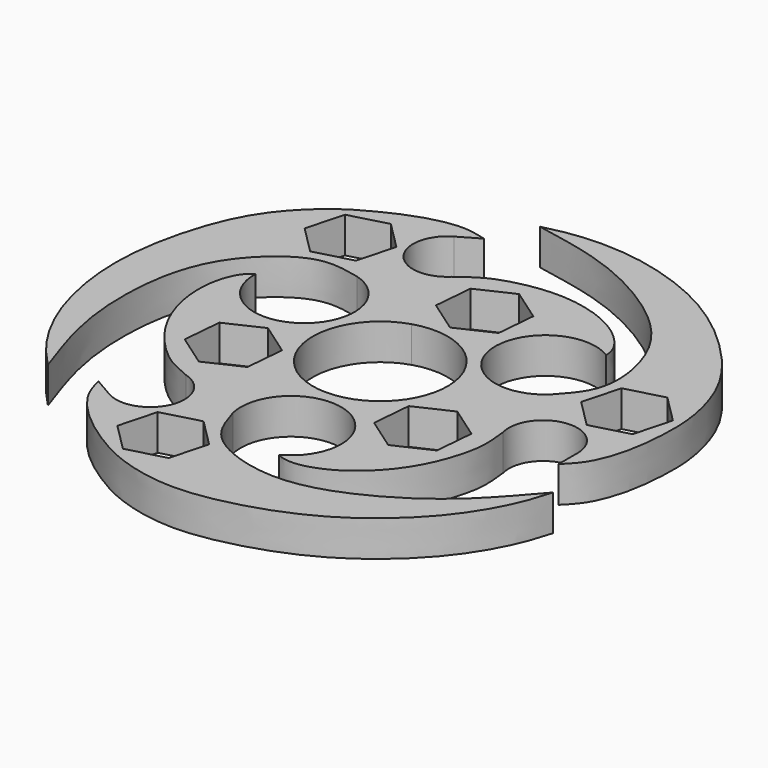
from build123d import *

# Parameters (mm, degrees)
F1_DEPTH = 5
F3_COUNT = 3
F5_DEPTH = 25
F6_DEPTH = 25


# Not quite as in the source:
# - a feature names something its author has since deleted; it is built from what else it names


with BuildPart() as f1:
    # F0 (on Top) → F1 (new body)
    with BuildSketch(Plane.XY):
        with BuildLine():
            ThreePointArc((19.3697792191, 5.4920897032), (7.5969915996, 9.8841483966), (18.2679687724, 16.5188265409))
            add(Edge.make_bspline(
                [(18.2679687724, 16.5188265409), (18.3496331671, 18.159304569), (15.0399422234, 22.4307572674), (5.8915424323, 25.1701629139), (-2.5645877448, 23.1556361007), (-4.2724416569, 21.9540160804), (-6.3755843906, 20.4204743588)],
                knots=[0, 0, 0, 0, 0.2303579847, 0.5244834011, 0.7878209886, 1, 1, 1, 1], degree=3))
            Line((-6.3755843906, 20.4204743588), (-2.8014574936, 8.9728387878))
            ThreePointArc((-2.8014574936, 8.9728387878), (6.3699775875, 6.9125527509), (9.1714350811, -2.0602860368))
            Line((9.1714350811, -2.0602860368), (20.8724397691, -4.6888186888))
            ThreePointArc((20.8724397691, -4.6888186888), (24.9046372172, 1.2367971287), (30.2800393035, -3.5041512456))
            Line((30.2800393035, -3.5041512456), (30.2800393035, -6.8021570911))
            add(Edge.make_bspline(
                [(-6.2640286051, 35.6329753995), (-4.879256488, 35.9717442203), (-1.585026432, 36.7719038353), (7.1656047644, 36.8306324291), (18.7097595399, 32.8325229218), (27.4190354107, 25.5475811449), (32.854692365, 18.5346088809), (34.9216993048, 10.9962495512), (34.9089688496, 5.8394018473), (34.4356780994, 0.7099122454), (32.81849257, -4.2517065064), (31.0670725646, -6.0125426883), (30.2800393035, -6.8021570911)],
                knots=[0, 0, 0, 0, 0.0814982335, 0.1926393238, 0.3258181235, 0.4537813969, 0.5666222077, 0.6709380758, 0.7568376371, 0.8431465468, 0.9290374106, 1, 1, 1, 1], degree=3))
            add(Edge.make_bspline(
                [(19.3697792191, 5.4920897032), (21.2657632456, 7.5222061316), (23.8510672601, 10.7996552166), (21.6544956387, 21.7849070989), (13.3248656234, 29.1499061822), (3.6795158583, 33.8104137468), (-3.1026823793, 35.0098141612), (-6.2640286051, 35.6329753995)],
                knots=[0, 0, 0, 0, 0.167152102, 0.3700687673, 0.5845137295, 0.7956301076, 1, 1, 1, 1], degree=3))
        make_face()
    extrude(amount=F1_DEPTH)

    # F3: F1 ×3 about axis
    f3_axis = Axis((0, 0, 27.9298778623), (0, 0, 1))


with BuildPart() as f1_1:
    add(f1.part)
    for i in range(1, F3_COUNT):
        add(f1.part.rotate(f3_axis, i * 360 / F3_COUNT))

    # F4 (on face) → F5 (cut)
    with BuildSketch(Plane.XY.offset(5)):
        Polygon((-3.5056654712, 14.0841332571), (0.9587131702, 10.958141679), (5.8980906096, 13.2614112055), (6.3730894075, 18.6906723101), (1.9087107662, 21.8166638882), (-3.0306666732, 19.5133943617), align=None)
        Polygon((13.0000523306, -14.8645934826), (17.9394297699, -12.5613239561), (18.4144285679, -7.1320628515), (13.9500499265, -4.0060712734), (9.0106724872, -6.3093407999), (8.5356736892, -11.7386019045), align=None)
        Polygon((-19.3731417381, -3.8260788275), (-19.8481405361, -9.2553399321), (-15.3837618947, -12.3813315102), (-10.4443844554, -10.0780619837), (-9.9693856574, -4.6488008791), (-14.4337642988, -1.522809301), align=None)
    extrude(amount=-F5_DEPTH, mode=Mode.SUBTRACT)

    # F4 (on face) → F6 (cut)
    with BuildSketch(Plane.XY.offset(5)):
        Polygon((-19.322068234, 25.9969277831), (-24.5863639873, 24.5863639873), (-25.9969277831, 19.322068234), (-22.1431958256, 15.4683362766), (-16.8789000724, 16.8789000724), (-15.4683362766, 22.1431958256), align=None)
        Polygon((32.1750339975, 3.7349380528), (33.5855977933, 8.999233806), (29.7318658359, 12.8529657635), (24.4675700826, 11.4424019677), (23.0570062868, 6.1781062144), (26.9107382443, 2.324374257), align=None)
        Polygon((-12.8529657635, -29.7318658359), (-8.999233806, -33.5855977933), (-3.7349380528, -32.1750339975), (-2.324374257, -26.9107382443), (-6.1781062144, -23.0570062868), (-11.4424019677, -24.4675700826), align=None)
    extrude(amount=-F6_DEPTH, mode=Mode.SUBTRACT)


solid = f1_1.part
